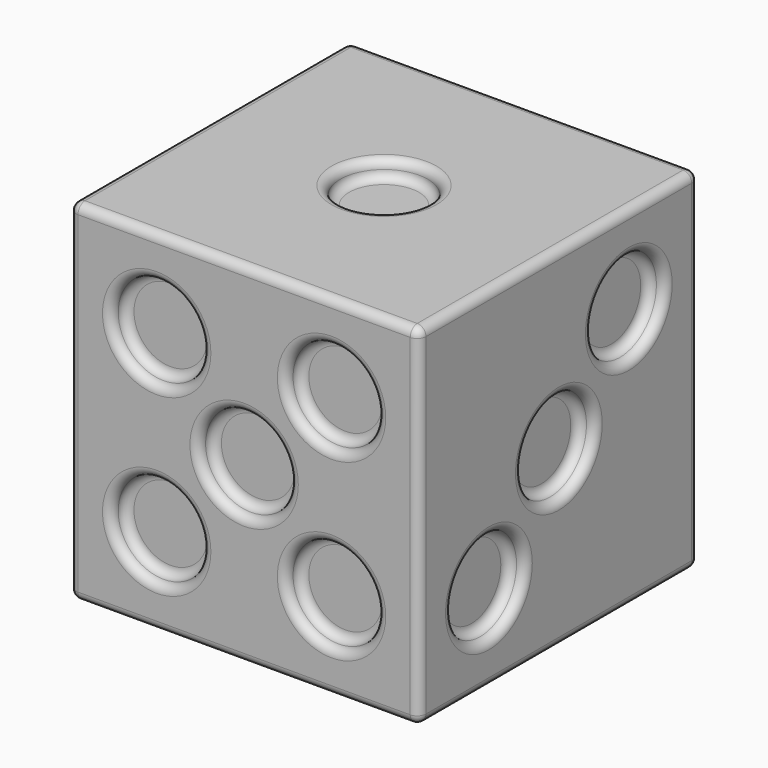
from build123d import *

# Parameters (mm, degrees)
F0_W      = 20
F0_H      = 20
F1_DEPTH  = 20
F2_R      = 2.6
F3_DEPTH  = 1
F4_R      = 0.49999
F5_R      = 2.6
F6_DEPTH  = 1
F7_R      = 0.49999
F8_R      = 2.5
F9_DEPTH  = 1
F10_R     = 0.49999
F11_R     = 2.6
F12_DEPTH = 1
F13_R     = 0.49999
F14_R     = 2.6
F15_DEPTH = 1
F16_R     = 0.49999
F17_R     = 2.6
F18_DEPTH = 1
F19_R     = 0.49999
F20_R     = 0.5


# Not quite as in the source:
# - a fillet or chamfer is up to 0.001 mm smaller than in the source, because OpenCascade refuses the exact size


with BuildPart() as f1:
    # F0 (on Front) → F1 (new body)
    with BuildSketch(Plane.XZ):
        with Locations((10, 10)):
            Rectangle(F0_W, F0_H)
    extrude(amount=F1_DEPTH)

    # F2 (on face) → F3 (cut)
    with BuildSketch(Plane.XZ.offset(20)):
        with Locations((5, 15)):
            Circle(F2_R)
        with Locations((5, 5)):
            Circle(F2_R)
        with Locations((10, 10)):
            Circle(F2_R)
        with Locations((15, 5)):
            Circle(F2_R)
        with Locations((15, 15)):
            Circle(F2_R)
    extrude(amount=-F3_DEPTH, mode=Mode.SUBTRACT)

    # F4 (radius 0.5 in the source; OpenCascade refuses exactly that, so slightly less here)
    f4_edges = [f1.edges().sort_by_distance(p)[0] for p in [
        (7.4, -20, 10),
        (7.4, -19, 10),
        (2.4, -20, 5),
        (2.4, -19, 5),
        (12.4, -20, 5),
        (12.4, -19, 5),
        (12.4, -19, 15),
        (12.4, -20, 15),
        (2.4, -20, 15),
        (2.4, -19, 15),
    ]]
    fillet(f4_edges, radius=F4_R)

    # F5 (on face) → F6 (cut)
    with BuildSketch(Plane(origin=(0, 0, 0), x_dir=(-1, 0, 0), z_dir=(0, 1, 0))):
        with Locations((-15, 15)):
            Circle(F5_R)
        with Locations((-5, 5)):
            Circle(F5_R)
    extrude(amount=-F6_DEPTH, mode=Mode.SUBTRACT)

    # F7 (radius 0.5 in the source; OpenCascade refuses exactly that, so slightly less here)
    f7_edges = [f1.edges().sort_by_distance(p)[0] for p in [
        (17.6, 0, 15),
        (17.6, -1, 15),
        (7.6, 0, 5),
        (7.6, -1, 5),
    ]]
    fillet(f7_edges, radius=F7_R)

    # F8 (on face) → F9 (cut)
    with BuildSketch(Plane.XY.offset(20)):
        with Locations((10, -10)):
            Circle(F8_R)
    extrude(amount=-F9_DEPTH, mode=Mode.SUBTRACT)

    # F10 (radius 0.5 in the source; OpenCascade refuses exactly that, so slightly less here)
    f10_edges = [f1.edges().sort_by_distance(p)[0] for p in [
        (7.5, -10, 20),
        (7.5, -10, 19),
    ]]
    fillet(f10_edges, radius=F10_R)

    # F11 (on face) → F12 (cut)
    with BuildSketch(Plane(origin=(0, 0, 0), x_dir=(1, 0, 0), z_dir=(0, 0, -1))):
        with Locations((5, 3.75)):
            Circle(F11_R)
        with Locations((5, 10)):
            Circle(F11_R)
        with Locations((5, 16.25)):
            Circle(F11_R)
        with Locations((15, 16.25)):
            Circle(F11_R)
        with Locations((15, 10)):
            Circle(F11_R)
        with Locations((15, 3.75)):
            Circle(F11_R)
    extrude(amount=-F12_DEPTH, mode=Mode.SUBTRACT)

    # F13 (radius 0.5 in the source; OpenCascade refuses exactly that, so slightly less here)
    f13_edges = [f1.edges().sort_by_distance(p)[0] for p in [
        (2.4, -16.25, 0),
        (2.4, -16.25, 1),
        (2.4, -10, 0),
        (2.4, -10, 1),
        (2.4, -3.75, 0),
        (2.4, -3.75, 1),
        (12.4, -16.25, 0),
        (12.4, -16.25, 1),
        (12.4, -10, 0),
        (12.4, -10, 1),
        (12.4, -3.75, 0),
        (12.4, -3.75, 1),
    ]]
    fillet(f13_edges, radius=F13_R)

    # F14 (on face) → F15 (cut)
    with BuildSketch(Plane.YZ.offset(20)):
        with Locations((-5, 15)):
            Circle(F14_R)
        with Locations((-10, 10)):
            Circle(F14_R)
        with Locations((-15, 5)):
            Circle(F14_R)
    extrude(amount=-F15_DEPTH, mode=Mode.SUBTRACT)

    # F16 (radius 0.5 in the source; OpenCascade refuses exactly that, so slightly less here)
    f16_edges = [f1.edges().sort_by_distance(p)[0] for p in [
        (20, -7.6, 15),
        (19, -7.6, 15),
        (20, -12.6, 10),
        (19, -12.6, 10),
        (19, -17.6, 5),
        (20, -17.6, 5),
    ]]
    fillet(f16_edges, radius=F16_R)

    # F17 (on face) → F18 (cut)
    with BuildSketch(Plane(origin=(0, 0, 0), x_dir=(0, -1, 0), z_dir=(-1, 0, 0))):
        with Locations((5, 15)):
            Circle(F17_R)
        with Locations((5, 5)):
            Circle(F17_R)
        with Locations((15, 5)):
            Circle(F17_R)
        with Locations((15, 15)):
            Circle(F17_R)
    extrude(amount=-F18_DEPTH, mode=Mode.SUBTRACT)

    # F19 (radius 0.5 in the source; OpenCascade refuses exactly that, so slightly less here)
    f19_edges = [f1.edges().sort_by_distance(p)[0] for p in [
        (0, -2.4, 15),
        (1, -2.4, 15),
        (0, -12.4, 15),
        (1, -12.4, 15),
        (0, -2.4, 5),
        (1, -2.4, 5),
        (0, -12.4, 5),
        (1, -12.4, 5),
    ]]
    fillet(f19_edges, radius=F19_R)

    # F20
    f20_edges = [f1.edges().sort_by_distance(p)[0] for p in [
        (0, -20, 10),
        (0, -10, 20),
        (10, -20, 20),
        (0, -10, 0),
        (10, -20, 0),
        (20, -20, 10),
        (20, -10, 0),
        (10, 0, 0),
        (20, 0, 10),
        (0, 0, 10),
        (10, 0, 20),
        (20, -10, 20),
    ]]
    fillet(f20_edges, radius=F20_R)


solid = f1.part
